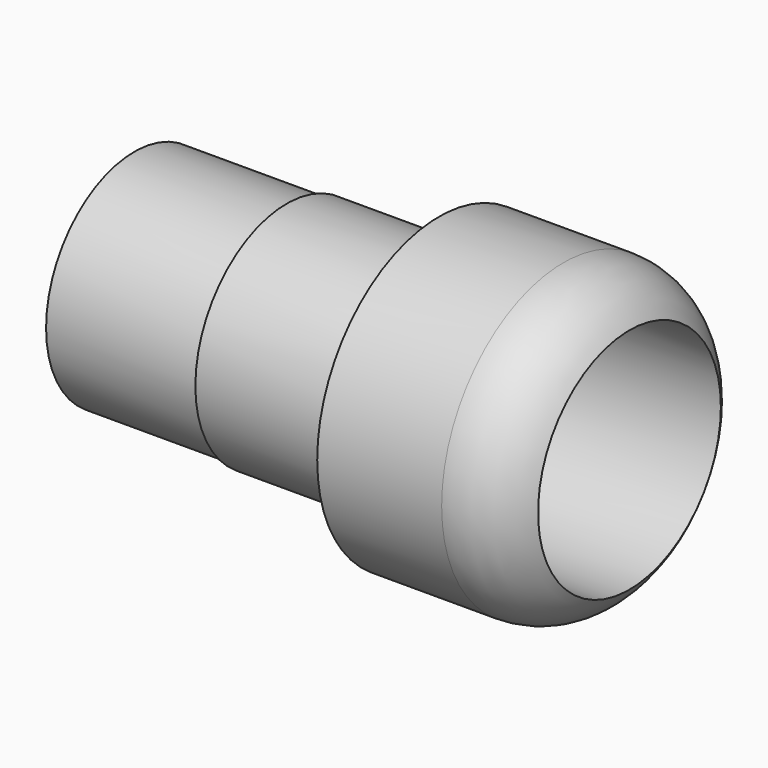
from build123d import *

# Parameters (mm, degrees)
F0_R     = 5.08
F1_DEPTH = 17.78
F2_R     = 5.08
F2_R_2   = 3.683
F3_DEPTH = 6.35
F4_R     = 5.08
F4_R_2   = 3.81
F5_DEPTH = 5.08
F6_R     = 3.81
F7_DEPTH = 5.08
F8_R     = 3.683
F9_DEPTH = 1.27


# Not quite as in the source:
# - a fillet or chamfer that OpenCascade refuses, or shapes differently, is made with other operations: its cross-section is extruded or revolved along the edge and cut away or added


with BuildPart() as f1:
    # F0 (on Right) → F1 (new body)
    with BuildSketch(Plane.YZ):
        Circle(F0_R)
    extrude(amount=F1_DEPTH)

    # F2 (on face) → F3 (cut)
    with BuildSketch(Plane(origin=(0, 0, 0), x_dir=(0, -1, 0), z_dir=(-1, 0, 0))):
        Circle(F2_R)
        Circle(F2_R_2, mode=Mode.SUBTRACT)
    extrude(amount=-F3_DEPTH, mode=Mode.SUBTRACT)

    # F4 (on face) → F5 (cut)
    with BuildSketch(Plane(origin=(6.35, 0, 0), x_dir=(0, -1, 0), z_dir=(-1, 0, 0))):
        Circle(F4_R)
        Circle(F4_R_2, mode=Mode.SUBTRACT)
    extrude(amount=-F5_DEPTH, mode=Mode.SUBTRACT)

    # F6 (on face) → F7 (cut)
    with BuildSketch(Plane.YZ.offset(17.78)):
        Circle(F6_R)
    extrude(amount=-F7_DEPTH, mode=Mode.SUBTRACT)

    # F8 (on face) → F9 (cut)
    with BuildSketch(Plane(origin=(0, 0, 0), x_dir=(0, -1, 0), z_dir=(-1, 0, 0))):
        Circle(F8_R)
    extrude(amount=-F9_DEPTH, mode=Mode.SUBTRACT)

    # F10: fillet of radius 2.54 on 1 edges, made by hand

    # F10_s1 → F10_t2 (revolve, cut)
    with BuildSketch(Plane.XY):
        with BuildLine():
            ThreePointArc((15.5802954744, 5.08), (16.8502954744, 4.7397045256), (17.78, 3.81))
            Line((17.78, 3.81), (17.78, 5.08))
            Line((17.78, 5.08), (15.5802954744, 5.08))
        make_face()
    revolve(axis=Axis((17.78, 0, 0), (1, 0, 0)), mode=Mode.SUBTRACT)


solid = f1.part
